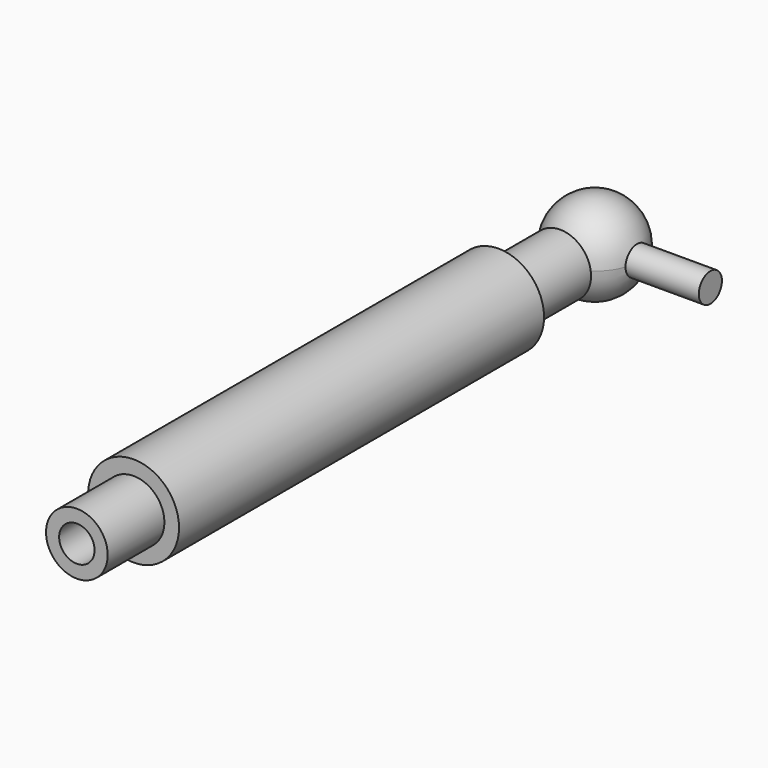
from build123d import *

# Parameters (mm, degrees)
F0_R      = 7.493
F1_DEPTH  = 75.184
F2_R      = 5.08
F3_DEPTH  = 12.7
F4_R      = 5.08
F5_DEPTH  = 11.684
F8_R      = 2.921
F9_DEPTH  = 82.55
F10_R     = 2.38125
F11_DEPTH = 19.05


with BuildPart() as f1:
    # F0 (on Front) → F1 (new body)
    with BuildSketch(Plane.XZ):
        Circle(F0_R)
    extrude(amount=F1_DEPTH)

    # F2 (on face) → F3 (join)
    with BuildSketch(Plane(origin=(0, 0, 0), x_dir=(-1, 0, 0), z_dir=(0, 1, 0))):
        Circle(F2_R)
    extrude(amount=F3_DEPTH)

    # F4 (on face) → F5 (join)
    with BuildSketch(Plane.XZ.offset(75.184)):
        Circle(F4_R)
    extrude(amount=F5_DEPTH)

    # F6 (on Right) → F7 (revolve)
    with BuildSketch(Plane.YZ):
        with BuildLine():
            ThreePointArc((19.812, -7.366), (25.0205485502, -5.2085485502), (27.178, 0))
            ThreePointArc((27.178, 0), (25.0205485502, 5.2085485502), (19.812, 7.366))
            Line((19.812, 7.366), (19.812, 0))
            Line((19.812, 0), (19.812, -7.366))
        make_face()
    revolve(axis=Axis((0, 19.812, 3.683), (0, 0, 1)))

    # F8 (on face) → F9 (cut)
    with BuildSketch(Plane.XZ.offset(86.868)):
        Circle(F8_R)
    extrude(amount=-F9_DEPTH, mode=Mode.SUBTRACT)

    # F10 (on Right) → F11 (join)
    with BuildSketch(Plane.YZ):
        with Locations((19.812, 0)):
            Circle(F10_R)
    extrude(amount=F11_DEPTH)


solid = f1.part
